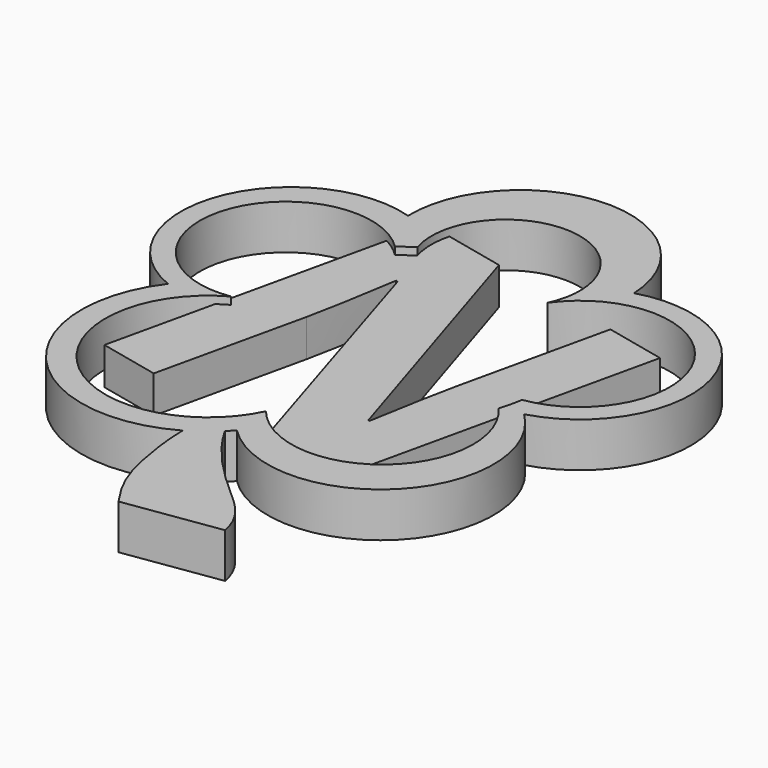
from build123d import *

# Parameters (mm, degrees)
F1_DEPTH     = 6
F2_TEXT_SIZE = 61.1111111111
F3_DEPTH     = 5
F5_DEPTH     = 6


# Not quite as in the source:
# - Text() gives the source's letters only with a copy of the font that has no kerning and outlines rounded to 1/6400 em; it was checked with that copy


with BuildPart() as f1:
    # F0 (on Top) → F1 (new body)
    with BuildSketch(Plane.XY):
        with BuildLine():
            ThreePointArc((1.6673808799, -29.7139173041), (23.1850945699, -29.5749271886), (22.8966183656, -8.0586983793))
            ThreePointArc((22.8966183656, -8.0586983793), (33.2353404975, 10.3772078334), (14.7383028598, 20.6061575272))
            ThreePointArc((14.7383028598, 20.6061575272), (-0.5422741015, 34.6683344622), (-14.7485770789, 19.5216579904))
            ThreePointArc((-14.7485770789, 19.5216579904), (-33.0751514911, 10.4262485912), (-24.7458583691, -8.260984428))
            ThreePointArc((-24.7458583691, -8.260984428), (-21.8728891632, -31.7104282976), (1.6673808799, -29.7139173041))
        make_face()
        with BuildLine():
            ThreePointArc((-17.7722622748, -6.3643103032), (-30.5378118713, 8.5725271944), (-11.4454952898, 13.21492081))
            ThreePointArc((-11.4454952898, 13.21492081), (-10.5044629037, 13.9114211501), (-9.5243262272, 14.5517232435))
            ThreePointArc((-9.5243262272, 14.5517232435), (0.7070180513, 27.4148238886), (9.0143377657, 13.2328563553))
            ThreePointArc((9.0143377657, 13.2328563553), (29.1707829708, 12.6569934488), (20.7050263405, -5.6445055627))
            ThreePointArc((20.7050263405, -5.6445055627), (20.4012743714, -7.1771207511), (19.9789278658, -8.6813807033))
            ThreePointArc((19.9789278658, -8.6813807033), (18.6903707294, -26.0549407684), (1.3443910375, -24.4369304603))
            ThreePointArc((1.3443910375, -24.4369304603), (-20.6368852086, -28.5412285703), (-17.7722622748, -6.3643103032))
        make_face(mode=Mode.SUBTRACT)
    extrude(amount=F1_DEPTH)

    # F2 (on Top) → F3 (join)
    with BuildSketch(Plane.XY):
        with Locations(Location((-27.8331898696, -20.5514687923), (0, 0, -12.6768965308))):
            Text('N', F2_TEXT_SIZE, font='Open Sans', font_style=FontStyle.BOLD, text_align=(TextAlign.LEFT, TextAlign.BOTTOM))
    extrude(amount=F3_DEPTH)

    # F4 (on Top) → F5 (join)
    with BuildSketch(Plane.XY):
        with BuildLine():
            add(Edge.make_bspline(
                [(2.0749992914, -50.0855937451), (0.2934038685, -47.5096098905), (-2.016602041, -43.3505263066), (-3.5319040535, -28.8335456103), (-0.9844063736, -29.824502245), (0, -29.1160250242)],
                knots=[0, 0, 0, 0, 0.3719534654, 0.8027362586, 1, 1, 1, 1], degree=3))
            Line((2.0749992914, -50.0855937451), (14.8857654416, -48.1903749471))
            add(Edge.make_bspline(
                [(14.8857654416, -48.1903749471), (14.1366781542, -44.4330575724), (8.4661418745, -40.3201932227), (2.0017706882, -33.3721849844), (0, -29.1160250242)],
                knots=[0, 0, 0, 0, 0.4605649299, 1, 1, 1, 1], degree=3))
        make_face()
    extrude(amount=F5_DEPTH)


solid = f1.part
